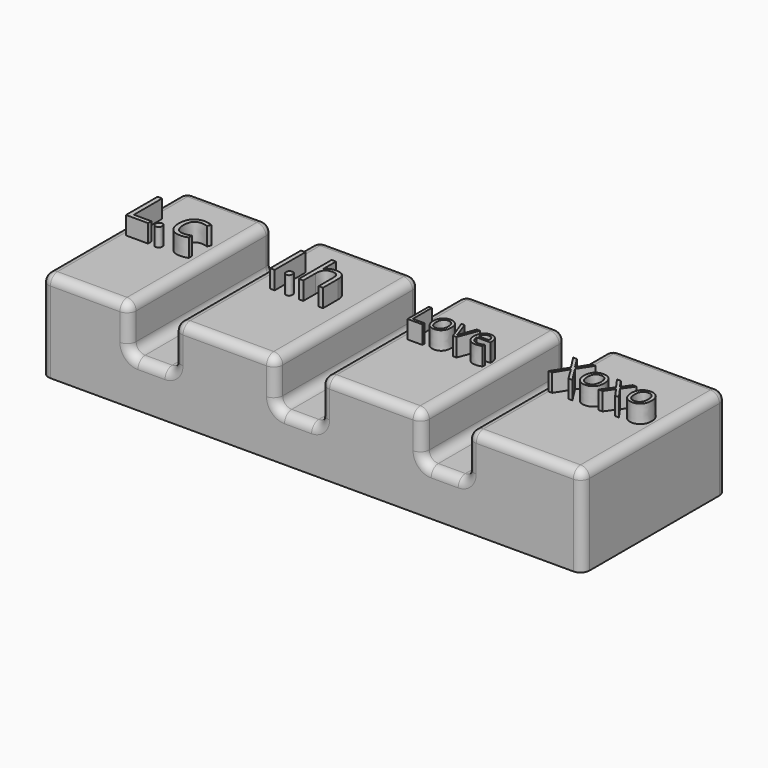
from build123d import *

# Parameters (mm, degrees)
F0_W         = 76.2
F0_H         = 25.4
F1_DEPTH     = 12.7
F2_W         = 6.35
F2_H         = 12.7
F3_DEPTH     = 25.401
F4_R         = 1.27
F5_T         = -2.54
F6_TEXT_SIZE = 7.7876003666
F10_DEPTH    = 2.54
F7_TEXT_SIZE = 7.5894692499
F11_DEPTH    = 2.54
F8_TEXT_SIZE = 5.2119040691
F12_DEPTH    = 2.54
F9_TEXT_SIZE = 5.9015207482
F13_DEPTH    = 2.54


# Not quite as in the source:
# - Text() gives the source's letters only with a copy of the font that has no kerning and outlines rounded to 1/6400 em; it was checked with that copy


with BuildPart() as f1:
    # F0 (on Top) → F1 (new body)
    with BuildSketch(Plane.XY):
        with Locations((1.9438185591, 0)):
            Rectangle(F0_W, F0_H)
    extrude(amount=F1_DEPTH)

    # F2 (on face) → F3 (cut, through all)
    with BuildSketch(Plane.XZ.offset(12.7)):
        with Locations((20.6502, 12.7)):
            Rectangle(F2_W, F2_H)
        with Locations((-20.6502, 12.7)):
            Rectangle(F2_W, F2_H)
        with Locations((0, 12.7)):
            Rectangle(F2_W, F2_H)
    extrude(amount=-F3_DEPTH, mode=Mode.SUBTRACT)

    # F4
    f4_edges = [f1.edges().sort_by_distance(p)[0] for p in [
        (-29.990691, 12.7, 12.7),
        (-23.8252, 0, 12.7),
        (-29.990691, -12.7, 12.7),
        (-36.156181, 0, 12.7),
        (-10.3251, 12.7, 12.7),
        (-3.175, 0, 12.7),
        (-10.3251, -12.7, 12.7),
        (-17.4752, 0, 12.7),
        (10.3251, 12.7, 12.7),
        (17.4752, 0, 12.7),
        (10.3251, -12.7, 12.7),
        (3.175, 0, 12.7),
        (31.934509, 12.7, 12.7),
        (40.043819, 0, 12.7),
        (31.934509, -12.7, 12.7),
        (23.8252, 0, 12.7),
        (-20.6502, -12.7, 6.35),
        (-17.4752, 0, 6.35),
        (-20.6502, 12.7, 6.35),
        (-23.8252, 0, 6.35),
        (0, -12.7, 6.35),
        (3.175, 0, 6.35),
        (0, 12.7, 6.35),
        (-3.175, 0, 6.35),
        (20.6502, -12.7, 6.35),
        (23.8252, 0, 6.35),
        (20.6502, 12.7, 6.35),
        (17.4752, 0, 6.35),
        (40.043819, -12.7, 6.35),
        (40.043819, 12.7, 6.35),
        (-36.156181, 12.7, 6.35),
        (-36.156181, -12.7, 6.35),
        (-23.8252, 12.7, 9.525),
        (-17.4752, 12.7, 9.525),
        (-3.175, 12.7, 9.525),
        (3.175, 12.7, 9.525),
        (17.4752, 12.7, 9.525),
        (23.8252, 12.7, 9.525),
        (23.8252, -12.7, 9.525),
        (17.4752, -12.7, 9.525),
        (3.175, -12.7, 9.525),
        (-3.175, -12.7, 9.525),
        (-17.4752, -12.7, 9.525),
        (-23.8252, -12.7, 9.525),
    ]]
    fillet(f4_edges, radius=F4_R)

    # F5
    f5_openings = [f1.faces().sort_by_distance(p)[0] for p in [
        (1.943819, 0, 0),
    ]]
    offset(amount=F5_T, openings=f5_openings)

    # F6 (on face) → F10 (join)
    with BuildSketch(Plane.XY.offset(12.7)):
        with Locations((-35.163107099, 0)):
            Text('L.c', F6_TEXT_SIZE, font='Open Sans', text_align=(TextAlign.LEFT, TextAlign.BOTTOM))
    extrude(amount=F10_DEPTH)

    # F7 (on face) → F11 (join)
    with BuildSketch(Plane.XY.offset(12.7)):
        with Locations((-14.8311182857, 0)):
            Text('I.h', F7_TEXT_SIZE, font='Open Sans', text_align=(TextAlign.LEFT, TextAlign.BOTTOM))
    extrude(amount=F11_DEPTH)

    # F8 (on face) → F12 (join)
    with BuildSketch(Plane.XY.offset(12.7)):
        with Locations((4.7512264482, 0)):
            Text('Love', F8_TEXT_SIZE, font='Open Sans', text_align=(TextAlign.LEFT, TextAlign.BOTTOM))
    extrude(amount=F12_DEPTH)

    # F9 (on face) → F13 (join)
    with BuildSketch(Plane.XY.offset(12.7)):
        with Locations((25.0952, 0)):
            Text('Xoxo', F9_TEXT_SIZE, font='Open Sans', text_align=(TextAlign.LEFT, TextAlign.BOTTOM))
    extrude(amount=F13_DEPTH)


solid = f1.part
